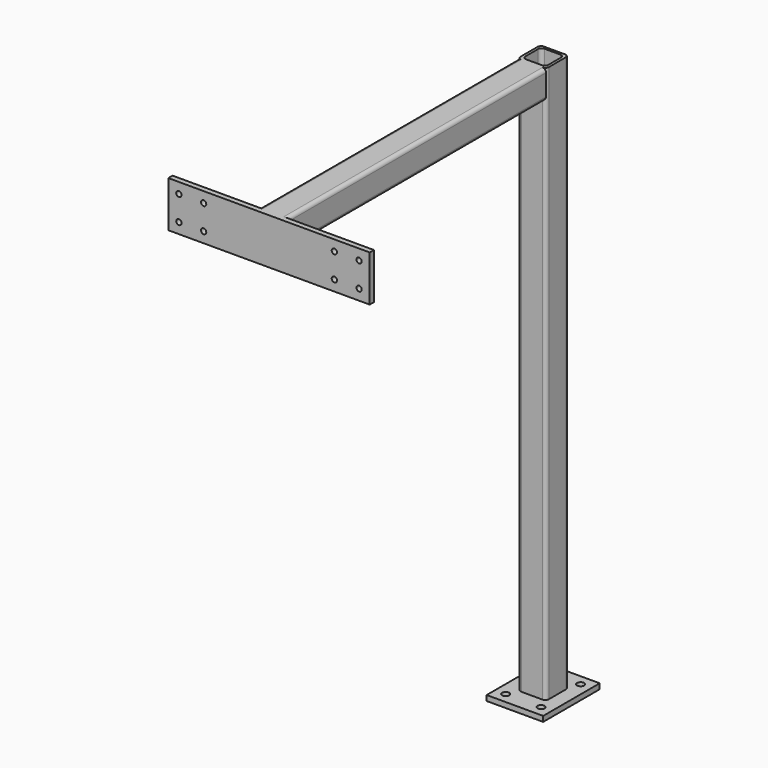
from build123d import *

# Parameters (mm, degrees)
F0_W     = 101.6
F0_H     = 127
F0_R     = 6.35
F1_DEPTH = 9.525
F4_DEPTH = 1000.125
F6_DEPTH = 581.025
F7_W     = 361.95
F7_H     = 82.55
F7_R     = 4.7625
F8_DEPTH = 9.525


# Not quite as in the source:
# - a length typed as a fraction of an inch, garbled in the dataset ("3 / 203.2 mm" for 3/8 in), is restored


with BuildPart() as f1:
    # F0 (on Top) → F1 (new body)
    with BuildSketch(Plane.XY):
        with Locations((50.8, 63.5)):
            Rectangle(F0_W, F0_H)
        with Locations((19.05, 19.05)):
            Circle(F0_R, mode=Mode.SUBTRACT)
        with Locations((82.55, 19.05)):
            Circle(F0_R, mode=Mode.SUBTRACT)
        with Locations((19.05, 107.95)):
            Circle(F0_R, mode=Mode.SUBTRACT)
        with Locations((82.55, 107.95)):
            Circle(F0_R, mode=Mode.SUBTRACT)
    extrude(amount=F1_DEPTH)

    # F3 (on offset) → F4 (join)
    with BuildSketch(Plane.XY.offset(9.525)):
        with BuildLine():
            Line((31.75, 38.1), (69.85, 38.1))
            ThreePointArc((69.85, 38.1), (74.3401280605, 39.9598719395), (76.2, 44.45))
            Line((76.2, 44.45), (76.2, 82.55))
            ThreePointArc((76.2, 82.55), (74.3401280605, 87.0401280605), (69.85, 88.9))
            Line((69.85, 88.9), (31.75, 88.9))
            ThreePointArc((31.75, 88.9), (27.2598719395, 87.0401280605), (25.4, 82.55))
            Line((25.4, 82.55), (25.4, 44.45))
            ThreePointArc((25.4, 44.45), (27.2598719395, 39.9598719395), (31.75, 38.1))
        make_face()
        with BuildLine():
            ThreePointArc((71.4375, 49.2125), (69.5776280605, 44.7223719395), (65.0875, 42.8625))
            Line((65.0875, 42.8625), (36.5125, 42.8625))
            ThreePointArc((36.5125, 42.8625), (32.0223719395, 44.7223719395), (30.1625, 49.2125))
            Line((30.1625, 49.2125), (30.1625, 77.7875))
            ThreePointArc((30.1625, 77.7875), (32.0223719395, 82.2776280605), (36.5125, 84.1375))
            Line((36.5125, 84.1375), (65.0875, 84.1375))
            ThreePointArc((65.0875, 84.1375), (69.5776280605, 82.2776280605), (71.4375, 77.7875))
            Line((71.4375, 77.7875), (71.4375, 49.2125))
        make_face(mode=Mode.SUBTRACT)
    extrude(amount=F4_DEPTH)

    # F5 (on face) → F6 (join)
    with BuildSketch(Plane.XZ.offset(-38.1)):
        with BuildLine():
            Line((31.75, 958.85), (69.85, 958.85))
            ThreePointArc((69.85, 958.85), (74.3401280605, 960.7098719395), (76.2, 965.2))
            Line((76.2, 965.2), (76.2, 1003.3))
            ThreePointArc((76.2, 1003.3), (74.3401280605, 1007.7901280605), (69.85, 1009.65))
            Line((69.85, 1009.65), (31.75, 1009.65))
            ThreePointArc((31.75, 1009.65), (27.2598719395, 1007.7901280605), (25.4, 1003.3))
            Line((25.4, 1003.3), (25.4, 965.2))
            ThreePointArc((25.4, 965.2), (27.2598719395, 960.7098719395), (31.75, 958.85))
        make_face()
        with BuildLine():
            ThreePointArc((71.4375, 969.9625), (69.5776280605, 965.4723719395), (65.0875, 963.6125))
            Line((65.0875, 963.6125), (36.5125, 963.6125))
            ThreePointArc((36.5125, 963.6125), (32.0223719395, 965.4723719395), (30.1625, 969.9625))
            Line((30.1625, 969.9625), (30.1625, 998.5375))
            ThreePointArc((30.1625, 998.5375), (32.0223719395, 1003.0276280605), (36.5125, 1004.8875))
            Line((36.5125, 1004.8875), (65.0875, 1004.8875))
            ThreePointArc((65.0875, 1004.8875), (69.5776280605, 1003.0276280605), (71.4375, 998.5375))
            Line((71.4375, 998.5375), (71.4375, 969.9625))
        make_face(mode=Mode.SUBTRACT)
    extrude(amount=F6_DEPTH)

    # F7 (on face) → F8 (join)
    with BuildSketch(Plane.XZ.offset(542.925)):
        with Locations((50.8, 968.375)):
            Rectangle(F7_W, F7_H)
        with Locations((-111.125, 946.15)):
            Circle(F7_R, mode=Mode.SUBTRACT)
        with Locations((-66.675, 946.15)):
            Circle(F7_R, mode=Mode.SUBTRACT)
        with Locations((168.275, 946.15)):
            Circle(F7_R, mode=Mode.SUBTRACT)
        with Locations((212.725, 946.15)):
            Circle(F7_R, mode=Mode.SUBTRACT)
        with Locations((-111.125, 990.6)):
            Circle(F7_R, mode=Mode.SUBTRACT)
        with Locations((-66.675, 990.6)):
            Circle(F7_R, mode=Mode.SUBTRACT)
        with Locations((168.275, 990.6)):
            Circle(F7_R, mode=Mode.SUBTRACT)
        with Locations((212.725, 990.6)):
            Circle(F7_R, mode=Mode.SUBTRACT)
    extrude(amount=F8_DEPTH)


solid = f1.part
